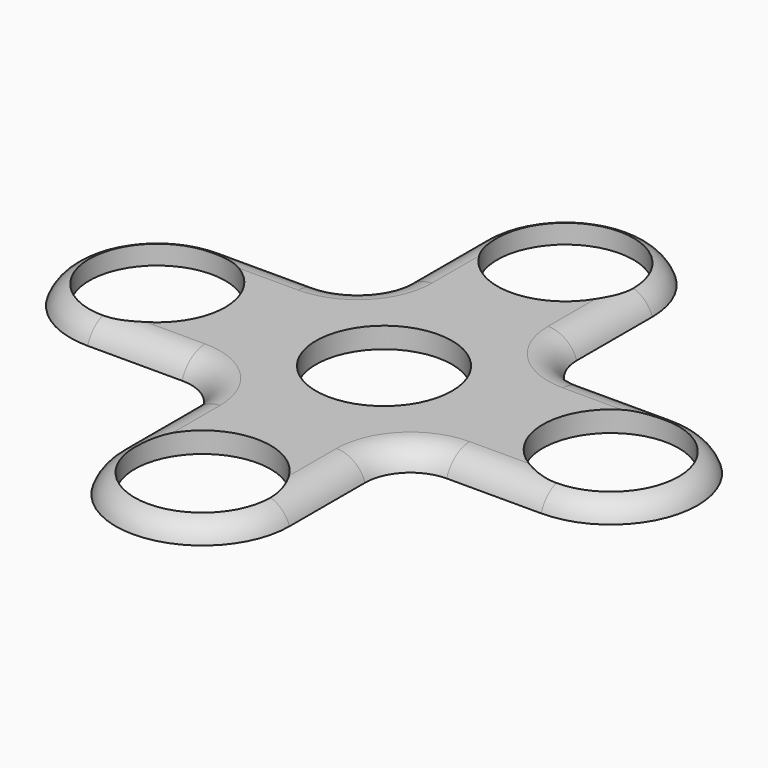
from build123d import *

# Parameters (mm, degrees)
F0_R         = 11.43
F0_R_2       = 14.605
F1_DEPTH     = 3.4925
F2_T1_DEPTH  = 15.875
F2_T3_DEPTH  = 15.875
F2_T5_DEPTH  = 15.875
F2_T7_DEPTH  = 15.875
F2_T10_ANGLE = 180
F2_T12_ANGLE = 90
F2_T14_ANGLE = 180
F2_T16_ANGLE = 90
F2_T18_ANGLE = 180
F2_T20_ANGLE = 90
F2_T22_ANGLE = 180
F2_T24_ANGLE = 90


# Not quite as in the source:
# - a fillet or chamfer that OpenCascade refuses, or shapes differently, is made with other operations: its cross-section is extruded or revolved along the edge and cut away or added


with BuildPart() as f1:
    # F0 (on Top) → F1 (new body)
    with BuildSketch(Plane.XY):
        with BuildLine():
            ThreePointArc((-14.605, 38.1), (0, 23.495), (14.605, 38.1))
            ThreePointArc((14.605, 38.1), (0, 52.705), (-14.605, 38.1))
        make_face()
        with Locations((0, 38.1)):
            Circle(F0_R, mode=Mode.SUBTRACT)
        with BuildLine():
            Line((14.605, 22.225), (14.605, 38.1))
            ThreePointArc((14.605, 38.1), (0, 23.495), (-14.605, 38.1))
            Line((-14.605, 38.1), (-14.605, 22.225))
            ThreePointArc((-14.605, 22.225), (-16.8368463274, 16.8368463274), (-22.225, 14.605))
            Line((-22.225, 14.605), (-38.1, 14.605))
            ThreePointArc((-38.1, 14.605), (-27.7727054608, 10.3272945392), (-23.495, 0))
            ThreePointArc((-23.495, 0), (-27.7727054608, -10.3272945392), (-38.1, -14.605))
            Line((-38.1, -14.605), (-22.225, -14.605))
            ThreePointArc((-22.225, -14.605), (-16.8368463274, -16.8368463274), (-14.605, -22.225))
            Line((-14.605, -22.225), (-14.605, -38.1))
            ThreePointArc((-14.605, -38.1), (0, -23.495), (14.605, -38.1))
            Line((14.605, -38.1), (14.605, -22.225))
            ThreePointArc((14.605, -22.225), (16.8368463274, -16.8368463274), (22.225, -14.605))
            Line((22.225, -14.605), (38.1, -14.605))
            ThreePointArc((38.1, -14.605), (23.495, 0), (38.1, 14.605))
            Line((38.1, 14.605), (22.225, 14.605))
            ThreePointArc((22.225, 14.605), (16.8368463274, 16.8368463274), (14.605, 22.225))
        make_face()
        Circle(F0_R_2, mode=Mode.SUBTRACT)
        with BuildLine():
            ThreePointArc((52.705, 0), (48.4272945392, 10.3272945392), (38.1, 14.605))
            ThreePointArc((38.1, 14.605), (23.495, 0), (38.1, -14.605))
            ThreePointArc((38.1, -14.605), (48.4272945392, -10.3272945392), (52.705, 0))
        make_face()
        with Locations((38.1, 0)):
            Circle(F0_R, mode=Mode.SUBTRACT)
        with BuildLine():
            ThreePointArc((-23.495, 0), (-27.7727054608, 10.3272945392), (-38.1, 14.605))
            ThreePointArc((-38.1, 14.605), (-52.705, 0), (-38.1, -14.605))
            ThreePointArc((-38.1, -14.605), (-27.7727054608, -10.3272945392), (-23.495, 0))
        make_face()
        with Locations((-38.1, 0)):
            Circle(F0_R, mode=Mode.SUBTRACT)
        with BuildLine():
            ThreePointArc((-14.605, -38.1), (0, -52.705), (14.605, -38.1))
            ThreePointArc((14.605, -38.1), (0, -23.495), (-14.605, -38.1))
        make_face()
        with Locations((0, -38.1)):
            Circle(F0_R, mode=Mode.SUBTRACT)
        Circle(F0_R_2)
        Circle(F0_R, mode=Mode.SUBTRACT)
    extrude(amount=F1_DEPTH)

    # F2: fillet of radius 5.08 on 1 edges, made by hand

    # F2_s2 → F2_t1 (cut)
    with BuildSketch(Plane.XZ.offset(22.225)):
        with BuildLine():
            ThreePointArc((-14.605, 0), (-12.7578317887, 2.5277703435), (-9.7794177812, 3.4925))
            Line((-9.7794177812, 3.4925), (-14.605, 3.4925))
            Line((-14.605, 3.4925), (-14.605, 0))
        make_face()
        with BuildLine():
            ThreePointArc((14.605, 0), (12.7578317887, 2.5277703435), (9.7794177812, 3.4925))
            Line((9.7794177812, 3.4925), (14.605, 3.4925))
            Line((14.605, 3.4925), (14.605, 0))
        make_face()
    extrude(amount=F2_T1_DEPTH, mode=Mode.SUBTRACT)

    # F2_s4 → F2_t3 (cut)
    with BuildSketch(Plane.YZ.offset(22.225)):
        with BuildLine():
            ThreePointArc((-14.605, 0), (-12.7578317887, 2.5277703435), (-9.7794177812, 3.4925))
            Line((-9.7794177812, 3.4925), (-14.605, 3.4925))
            Line((-14.605, 3.4925), (-14.605, 0))
        make_face()
        with BuildLine():
            ThreePointArc((14.605, 0), (12.7578317887, 2.5277703435), (9.7794177812, 3.4925))
            Line((9.7794177812, 3.4925), (14.605, 3.4925))
            Line((14.605, 3.4925), (14.605, 0))
        make_face()
    extrude(amount=F2_T3_DEPTH, mode=Mode.SUBTRACT)

    # F2_s6 → F2_t5 (cut)
    with BuildSketch(Plane.XZ.offset(-38.1)):
        with BuildLine():
            ThreePointArc((14.605, 0), (12.7578317887, 2.5277703435), (9.7794177812, 3.4925))
            Line((9.7794177812, 3.4925), (14.605, 3.4925))
            Line((14.605, 3.4925), (14.605, 0))
        make_face()
        with BuildLine():
            ThreePointArc((-14.605, 0), (-12.7578317887, 2.5277703435), (-9.7794177812, 3.4925))
            Line((-9.7794177812, 3.4925), (-14.605, 3.4925))
            Line((-14.605, 3.4925), (-14.605, 0))
        make_face()
    extrude(amount=F2_T5_DEPTH, mode=Mode.SUBTRACT)

    # F2_s8 → F2_t7 (cut)
    with BuildSketch(Plane.YZ.offset(-38.1)):
        with BuildLine():
            ThreePointArc((14.605, 0), (12.7578317887, 2.5277703435), (9.7794177812, 3.4925))
            Line((9.7794177812, 3.4925), (14.605, 3.4925))
            Line((14.605, 3.4925), (14.605, 0))
        make_face()
        with BuildLine():
            ThreePointArc((-14.605, 0), (-12.7578317887, 2.5277703435), (-9.7794177812, 3.4925))
            Line((-9.7794177812, 3.4925), (-14.605, 3.4925))
            Line((-14.605, 3.4925), (-14.605, 0))
        make_face()
    extrude(amount=F2_T7_DEPTH, mode=Mode.SUBTRACT)

    # F2_s9 → F2_t10 (revolve, cut)
    with BuildSketch(Plane.XZ.offset(38.1)):
        with BuildLine():
            ThreePointArc((-14.605, 0), (-12.7578317887, 2.5277703435), (-9.7794177812, 3.4925))
            Line((-9.7794177812, 3.4925), (-14.605, 3.4925))
            Line((-14.605, 3.4925), (-14.605, 0))
        make_face()
    revolve(axis=Axis((0, -38.1, 3.4925), (0, 0, 1)), revolution_arc=F2_T10_ANGLE, mode=Mode.SUBTRACT)

    # F2_s11 → F2_t12 (revolve, cut)
    with BuildSketch(Plane.XZ.offset(22.225)):
        with BuildLine():
            ThreePointArc((14.605, 0), (12.7578317887, 2.5277703435), (9.7794177812, 3.4925))
            Line((9.7794177812, 3.4925), (14.605, 3.4925))
            Line((14.605, 3.4925), (14.605, 0))
        make_face()
    revolve(axis=Axis((22.225, -22.225, 3.4925), (0, 0, -1)), revolution_arc=F2_T12_ANGLE, mode=Mode.SUBTRACT)

    # F2_s13 → F2_t14 (revolve, cut)
    with BuildSketch(Plane.YZ.offset(38.1)):
        with BuildLine():
            ThreePointArc((-14.605, 0), (-12.7578317887, 2.5277703435), (-9.7794177812, 3.4925))
            Line((-9.7794177812, 3.4925), (-14.605, 3.4925))
            Line((-14.605, 3.4925), (-14.605, 0))
        make_face()
    revolve(axis=Axis((38.1, 0, 3.4925), (0, 0, 1)), revolution_arc=F2_T14_ANGLE, mode=Mode.SUBTRACT)

    # F2_s15 → F2_t16 (revolve, cut)
    with BuildSketch(Plane.YZ.offset(22.225)):
        with BuildLine():
            ThreePointArc((14.605, 0), (12.7578317887, 2.5277703435), (9.7794177812, 3.4925))
            Line((9.7794177812, 3.4925), (14.605, 3.4925))
            Line((14.605, 3.4925), (14.605, 0))
        make_face()
    revolve(axis=Axis((22.225, 22.225, 3.4925), (0, 0, -1)), revolution_arc=F2_T16_ANGLE, mode=Mode.SUBTRACT)

    # F2_s17 → F2_t18 (revolve, cut)
    with BuildSketch(Plane.XZ.offset(-38.1)):
        with BuildLine():
            ThreePointArc((14.605, 0), (12.7578317887, 2.5277703435), (9.7794177812, 3.4925))
            Line((9.7794177812, 3.4925), (14.605, 3.4925))
            Line((14.605, 3.4925), (14.605, 0))
        make_face()
    revolve(axis=Axis((0, 38.1, 3.4925), (0, 0, 1)), revolution_arc=F2_T18_ANGLE, mode=Mode.SUBTRACT)

    # F2_s19 → F2_t20 (revolve, cut)
    with BuildSketch(Plane.XZ.offset(-22.225)):
        with BuildLine():
            ThreePointArc((-14.605, 0), (-12.7578317887, 2.5277703435), (-9.7794177812, 3.4925))
            Line((-9.7794177812, 3.4925), (-14.605, 3.4925))
            Line((-14.605, 3.4925), (-14.605, 0))
        make_face()
    revolve(axis=Axis((-22.225, 22.225, 3.4925), (0, 0, -1)), revolution_arc=F2_T20_ANGLE, mode=Mode.SUBTRACT)

    # F2_s21 → F2_t22 (revolve, cut)
    with BuildSketch(Plane.YZ.offset(-38.1)):
        with BuildLine():
            ThreePointArc((14.605, 0), (12.7578317887, 2.5277703435), (9.7794177812, 3.4925))
            Line((9.7794177812, 3.4925), (14.605, 3.4925))
            Line((14.605, 3.4925), (14.605, 0))
        make_face()
    revolve(axis=Axis((-38.1, 0, 3.4925), (0, 0, 1)), revolution_arc=F2_T22_ANGLE, mode=Mode.SUBTRACT)

    # F2_s23 → F2_t24 (revolve, cut)
    with BuildSketch(Plane.YZ.offset(-22.225)):
        with BuildLine():
            ThreePointArc((-14.605, 0), (-12.7578317887, 2.5277703435), (-9.7794177812, 3.4925))
            Line((-9.7794177812, 3.4925), (-14.605, 3.4925))
            Line((-14.605, 3.4925), (-14.605, 0))
        make_face()
    revolve(axis=Axis((-22.225, -22.225, 3.4925), (0, 0, -1)), revolution_arc=F2_T24_ANGLE, mode=Mode.SUBTRACT)


solid = f1.part
